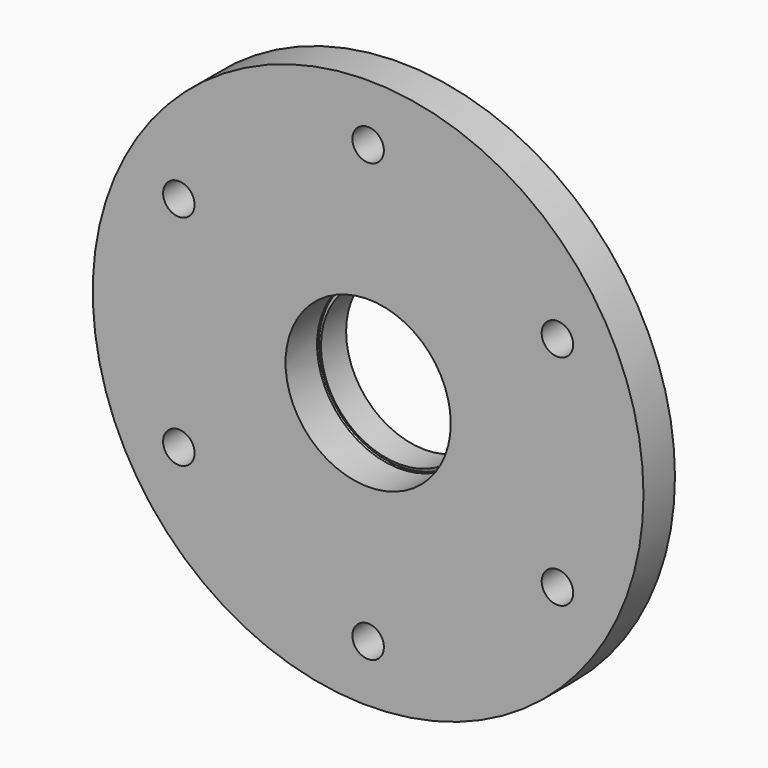
from build123d import *

# Parameters (mm, degrees)
F0_R     = 70
F0_R_2   = 4
F0_R_3   = 21
F1_DEPTH = 10
F2_R     = 21
F3_DEPTH = 8
F4_SIZE  = 1
F6_R     = 20
F7_DEPTH = 20


# Not quite as in the source:
# - a fillet or chamfer that OpenCascade refuses, or shapes differently, is made with other operations: its cross-section is extruded or revolved along the edge and cut away or added


with BuildPart() as f1:
    # F0 (on Front) → F1 (new body)
    with BuildSketch(Plane.XZ):
        Circle(F0_R)
        with Locations((-48.1207015613, -27.7825)):
            Circle(F0_R_2, mode=Mode.SUBTRACT)
        with Locations((0, -55.565)):
            Circle(F0_R_2, mode=Mode.SUBTRACT)
        with Locations((48.1207015613, -27.7825)):
            Circle(F0_R_2, mode=Mode.SUBTRACT)
        with Locations((-48.1207015613, 27.7825)):
            Circle(F0_R_2, mode=Mode.SUBTRACT)
        Circle(F0_R_3, mode=Mode.SUBTRACT)
        with Locations((48.1207015613, 27.7825)):
            Circle(F0_R_2, mode=Mode.SUBTRACT)
        with Locations((0, 55.565)):
            Circle(F0_R_2, mode=Mode.SUBTRACT)
    extrude(amount=F1_DEPTH)

    # F2 (on Front) → F3 (join)
    with BuildSketch(Plane.XZ):
        Circle(F2_R)
    extrude(amount=-F3_DEPTH)

    # F4
    f4_edges = [f1.edges().sort_by_distance(p)[0] for p in [
        (-21, 8, 0),
    ]]
    chamfer(f4_edges, length=F4_SIZE)

    # F5: fillet of radius 1 on 1 edges, made by hand

    # F5_s1 → F5_t2 (revolve, cut)
    with BuildSketch(Plane.XY):
        with BuildLine():
            ThreePointArc((21, 1), (20.7071067812, 0.2928932188), (20, 0))
            Line((20, 0), (21, 0))
            Line((21, 0), (21, 1))
        make_face()
    revolve(axis=Axis((0, 0, 0), (0, -1, 0)), mode=Mode.SUBTRACT)

    # F6 (on face) → F7 (cut)
    with BuildSketch(Plane(origin=(0, 8, 0), x_dir=(-1, 0, 0), z_dir=(0, 1, 0))):
        Circle(F6_R)
    extrude(amount=-F7_DEPTH, mode=Mode.SUBTRACT)


solid = f1.part
